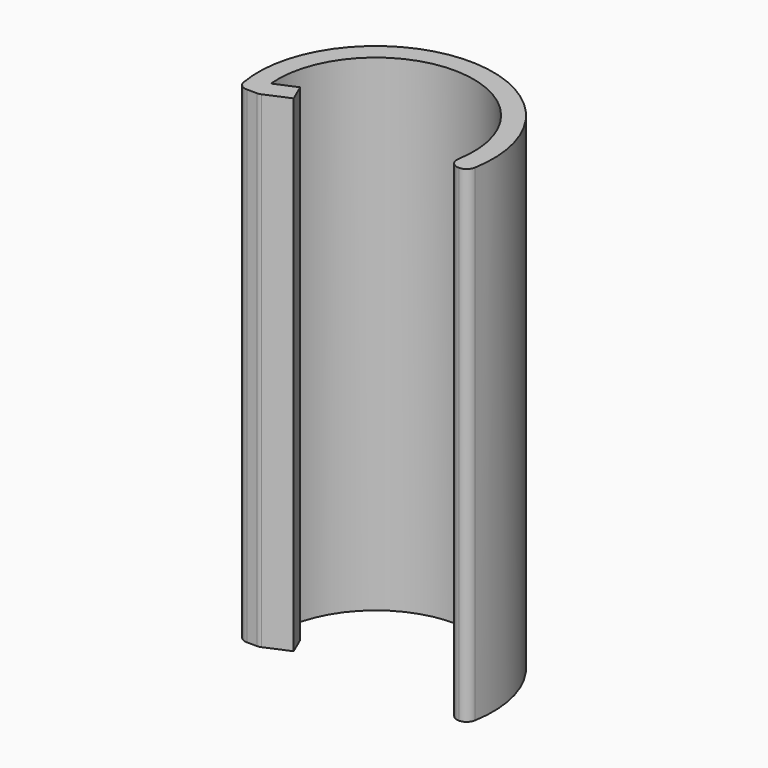
from build123d import *

# Parameters (mm, degrees)
F1_DEPTH = 40
F2_R     = 0.79999


# Not quite as in the source:
# - a fillet or chamfer is up to 0.001 mm smaller than in the source, because OpenCascade refuses the exact size


with BuildPart() as f1:
    # F0 (on Top) → F1 (new body)
    with BuildSketch(Plane.XY):
        with BuildLine():
            ThreePointArc((-8.0155554774, -0.7438886939), (0.8184709888, 8.008283539), (7.699350622, -2.35))
            Line((7.699350622, -2.35), (9.3594871654, -2.35))
            ThreePointArc((9.3594871654, -2.35), (0, 9.65), (-9.3594871654, -2.35))
            Line((-9.3594871654, -2.35), (-7.699350622, -2.35))
            Line((-7.699350622, -2.35), (-5.5929206907, -1.4413775962))
            Line((-5.5929206907, -1.4413775962), (-6.2266466845, 0.0277688788))
            Line((-6.2266466845, 0.0277688788), (-8.0155554774, -0.7438886939))
        make_face()
    extrude(amount=F1_DEPTH)

    # F2 (radius 0.8 in the source; OpenCascade refuses exactly that, so slightly less here)
    f2_edges = [f1.edges().sort_by_distance(p)[0] for p in [
        (-7.699351, -2.35, 20),
        (7.699351, -2.35, 20),
        (9.359487, -2.35, 20),
        (-9.359487, -2.35, 20),
    ]]
    fillet(f2_edges, radius=F2_R)


solid = f1.part
